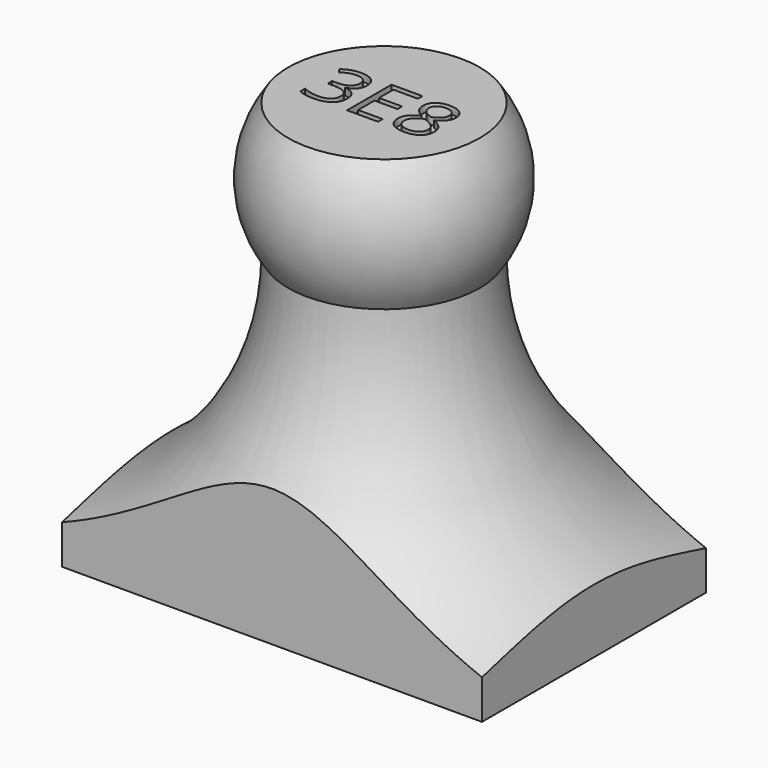
from build123d import *

# Parameters (mm, degrees)
F2_R         = 50
F2_W         = 60
F2_H         = 40
F3_DEPTH     = 60.0010001
F4_TEXT_SIZE = 11.1111111111
F5_DEPTH     = 1


# Not quite as in the source:
# - Text() gives the source's letters only with a copy of the font that has no kerning and outlines rounded to 1/6400 em; it was checked with that copy


with BuildPart() as f1:
    # F0 (on Front) → F1 (revolve)
    with BuildSketch(Plane.XZ):
        with BuildLine():
            Line((0, 60), (0, 0))
            Line((0, 0), (50, 0))
            Line((50, 0), (50, 2))
            ThreePointArc((50, 2), (24.0753831122, 14.3609595603), (13.6914541945, 41.1388067901))
            ThreePointArc((13.6914541945, 41.1388067901), (16.7508092139, 50.5694033951), (13.6914541945, 60))
            Line((13.6914541945, 60), (0, 60))
        make_face()
    revolve(axis=Axis((0, 0, 30), (0, 0, -1)))

    # F2 (on face) → F3 (cut, through all)
    with BuildSketch(Plane(origin=(0, 0, 0), x_dir=(1, 0, 0), z_dir=(0, 0, -1))):
        Circle(F2_R)
        Rectangle(F2_W, F2_H, mode=Mode.SUBTRACT)
    extrude(amount=-F3_DEPTH, mode=Mode.SUBTRACT)

    # F4 (on face) → F5 (cut)
    with BuildSketch(Plane.XY.offset(60)):
        with Locations((-9.5147569444, -4)):
            Text('3E8', F4_TEXT_SIZE, font='Open Sans', text_align=(TextAlign.LEFT, TextAlign.BOTTOM))
    extrude(amount=-F5_DEPTH, mode=Mode.SUBTRACT)


solid = f1.part
